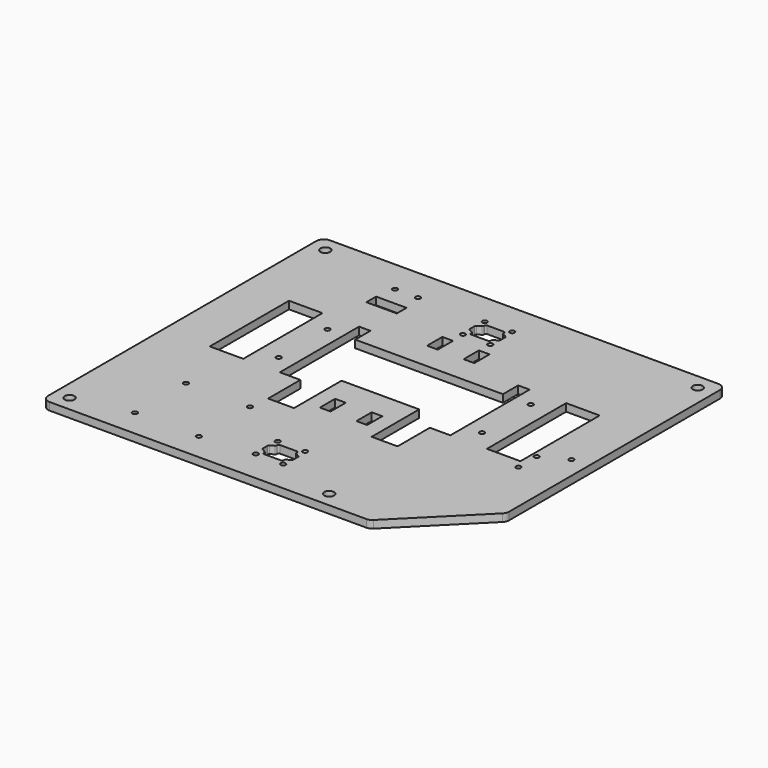
from build123d import *

# Parameters (mm, degrees)
F0_W      = 265
F0_H      = 230
F0_W_2    = 22
F0_H_2    = 65
F1_DEPTH  = 5
F2_D      = 3.2
F5_DEPTH  = 5
F6_D      = 3.2
F7_R      = 1
F8_W      = 7
F8_H      = 12.5
F9_DEPTH  = 5.001
F10_SIZE2 = 50
F10_SIZE  = 50
F12_D     = 6.4
F14_R     = 5
F16_D     = 3.2
F16_DEPTH = 5
F16_TIP   = 0.9613769904
F17_D     = 3.2
F17_DEPTH = 5
F17_TIP   = 0.9613769904
F18_R     = 1.6
F18_W     = 20
F18_H     = 8
F19_DEPTH = 25


# Not quite as in the source:
# - a pattern or mirror of a feature is missing from the dataset's text; its kind, count and spacing are read off the source's solid


with BuildPart() as f1:
    # F0 (on Top) → F1 (new body)
    with BuildSketch(Plane.XY):
        with Locations((0, -17)):
            Rectangle(F0_W, F0_H)
        with Locations((-91, 0)):
            Rectangle(F0_W_2, F0_H_2, mode=Mode.SUBTRACT)
        Polygon((56, 32.5), (56, -32.5), (42.5, -32.5), (42.5, -59), (25.5, -59), (25.5, -20), (-25.5, -20), (-25.5, -59), (-42.5, -59), (-42.5, -32.5), (-56, -32.5), (-56, 32.5), (-48.5, 32.5), (-48.5, 20), (48.5, 20), (48.5, 32.5), align=None, mode=Mode.SUBTRACT)
        with Locations((91, 0)):
            Rectangle(F0_W_2, F0_H_2, mode=Mode.SUBTRACT)
    extrude(amount=F1_DEPTH)

    # F2 (through all)
    with Locations(Plane(origin=(0, 0, 0), x_dir=(1, 0, 0), z_dir=(0, 0, -1))):
        with Locations((-66.75, -20), (-66.75, 20), (66.75, -20), (66.75, 20)):
            Hole(F2_D / 2)

    # F4 (on face) → F5 (cut, through all)
    with BuildSketch(Plane.XY.offset(5)):
        Polygon((-6.5, -108.5), (6.5, -108.5), (6.5, -106.5207259422), (10, -104.5), (10, -99.5), (6.5, -97.4792740578), (6.5, -95.5), (-6.5, -95.5), (-6.5, -97.4792740578), (-10, -99.5), (-10, -104.5), (-6.5, -106.5207259422), align=None)
    f5 = extrude(amount=-F5_DEPTH, mode=Mode.SUBTRACT)

    # F5_copies: F5 across plane
    add(f5.mirror(Plane.ZX.offset(-17)), mode=Mode.SUBTRACT)

    # F6 (through all)
    with Locations(Plane.XY.offset(5)):
        with Locations((-9, -93), (-9, -111), (9, -93), (9, -111)):
            f6 = Hole(F6_D / 2)

    # F6_copies: F6 across plane
    add(f6.mirror(Plane.ZX.offset(-17)), mode=Mode.SUBTRACT)

    # F7
    f7_edges = [f1.edges().sort_by_distance(p)[0] for p in [
        (-10, -99.5, 2.5),
        (-6.5, -97.479274, 2.5),
        (-6.5, -95.5, 2.5),
        (6.5, -95.5, 2.5),
        (6.5, -97.479274, 2.5),
        (10, -99.5, 2.5),
        (10, -104.5, 2.5),
        (6.5, -106.520726, 2.5),
        (6.5, -108.5, 2.5),
        (-6.5, -108.5, 2.5),
        (-6.5, -106.520726, 2.5),
        (-10, -104.5, 2.5),
        (-6.5, 72.520726, 2.5),
        (-6.5, 74.5, 2.5),
        (-10, 70.5, 2.5),
        (6.5, 74.5, 2.5),
        (-10, 65.5, 2.5),
        (6.5, 72.520726, 2.5),
        (-6.5, 63.479274, 2.5),
        (10, 70.5, 2.5),
        (-6.5, 61.5, 2.5),
        (10, 65.5, 2.5),
        (6.5, 61.5, 2.5),
        (6.5, 63.479274, 2.5),
    ]]
    fillet(f7_edges, radius=F7_R)

    # F8 (on face) → F9 (cut, through all)
    with BuildSketch(Plane.XY.offset(5)):
        with Locations((-12, -44)):
            Rectangle(F8_W, F8_H)
        with Locations((12, -44)):
            Rectangle(F8_W, F8_H)
        with Locations((-12, 44)):
            Rectangle(F8_W, F8_H)
        with Locations((12, 44)):
            Rectangle(F8_W, F8_H)
    extrude(amount=-F9_DEPTH, mode=Mode.SUBTRACT)

    # F10
    f10_edges = [f1.edges().sort_by_distance(p)[0] for p in [
        (132.5, -132, 2.5),
    ]]
    chamfer(f10_edges, length=F10_SIZE, length2=F10_SIZE2)

    # F12 (through all)
    with Locations(Plane(origin=(0, 0, 0), x_dir=(1, 0, 0), z_dir=(0, 0, -1))):
        with Locations((-122.5, -88), (-122.5, 122), (48, 122), (122, -88)):
            Hole(F12_D / 2)

    # F14
    f14_edges = [f1.edges().sort_by_distance(p)[0] for p in [
        (-132.5, -132, 2.5),
        (-132.5, 98, 2.5),
        (132.5, 98, 2.5),
        (132.5, -82, 2.5),
        (82.5, -132, 2.5),
    ]]
    fillet(f14_edges, radius=F14_R)

    # F16
    with Locations(Plane.XY.offset(5)):
        with Locations((105.3, -23.3), (105.3, -38.3), (121.3, -14.8)):
            Hole(F16_D / 2, depth=F16_DEPTH)
            with Locations((0, 0, -(F16_DEPTH + F16_TIP / 2))):  # 118° drill point
                Cone(0, F16_D / 2, F16_TIP, mode=Mode.SUBTRACT)

    # F17
    with Locations(Plane(origin=(0, 0, 0), x_dir=(1, 0, 0), z_dir=(0, 0, -1))):
        with Locations((-86, 72), (-86, 114), (-44, 72), (-44, 114)):
            Hole(F17_D / 2, depth=F17_DEPTH)
            with Locations((0, 0, -(F17_DEPTH + F17_TIP / 2))):  # 118° drill point
                Cone(0, F17_D / 2, F17_TIP, mode=Mode.SUBTRACT)

    # F18 (on Top) → F19 (cut)
    with BuildSketch(Plane.XY):
        with Locations((-67.5, 76.5)):
            Circle(F18_R)
        with Locations((-52.5, 76.5)):
            Circle(F18_R)
        with Locations((-60, 60)):
            Rectangle(F18_W, F18_H)
    extrude(amount=F19_DEPTH, mode=Mode.SUBTRACT)


solid = f1.part
